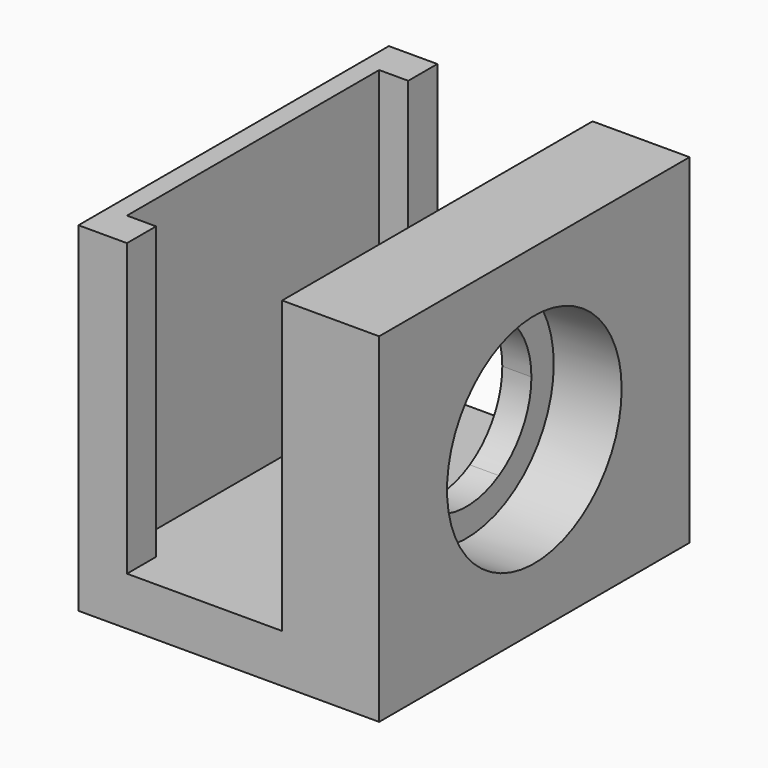
from build123d import *

# Parameters (mm, degrees)
F1_DEPTH = 20
F2_R     = 11.25
F3_DEPTH = 7
F4_R     = 6.75
F5_DEPTH = 5
F6_W     = 3
F6_H     = 32.5
F7_DEPTH = 30
F8_R     = 6.75
F9_DEPTH = 25


with BuildPart() as f1:
    # F0 (on Front) → F1 (new body, symmetric)
    with BuildSketch(Plane.XZ):
        Polygon((-25, 35), (-30, 35), (-30, 0), (1, 0), (1, 35), (-9, 35), (-9, 5), (-25, 5), align=None)
    extrude(amount=F1_DEPTH, both=True)

    # F2 (on face) → F3 (cut)
    with BuildSketch(Plane.YZ.offset(1)):
        with Locations((0, 17.5)):
            Circle(F2_R)
    extrude(amount=-F3_DEPTH, mode=Mode.SUBTRACT)

    # F4 (on face) → F5 (cut)
    with BuildSketch(Plane.YZ.offset(-6)):
        with Locations((0, 17.5)):
            Circle(F4_R)
    extrude(amount=-F5_DEPTH, mode=Mode.SUBTRACT)

    # F6 (on face) → F7 (cut)
    with BuildSketch(Plane.XY.offset(35)):
        with Locations((-26.5, 0)):
            Rectangle(F6_W, F6_H)
    extrude(amount=-F7_DEPTH, mode=Mode.SUBTRACT)

    # F8 (on face) → F9 (cut)
    with BuildSketch(Plane(origin=(-9, 0, 0), x_dir=(0, -1, 0), z_dir=(-1, 0, 0))):
        Polygon((4.1857894516, 24.75), (-4.1857894516, 24.75), (-8.3715789032, 17.5), (-4.1857894516, 10.25), (4.1857894516, 10.25), (8.3715789032, 17.5), align=None)
        with Locations((0, 17.5)):
            Circle(F8_R, mode=Mode.SUBTRACT)
        with Locations((0, 17.5)):
            Circle(F8_R)
        with BuildLine():
            ThreePointArc((4.1857894516, 24.75), (0, 25.8715789032), (-4.1857894516, 24.75))
            Line((-4.1857894516, 24.75), (4.1857894516, 24.75))
        make_face()
        with BuildLine():
            Line((-8.3715789032, 17.5), (-4.1857894516, 24.75))
            ThreePointArc((-4.1857894516, 24.75), (-7.25, 21.6857894516), (-8.3715789032, 17.5))
        make_face()
        with BuildLine():
            ThreePointArc((8.3715789032, 17.5), (7.25, 21.6857894516), (4.1857894516, 24.75))
            Line((4.1857894516, 24.75), (8.3715789032, 17.5))
        make_face()
        with BuildLine():
            Line((-4.1857894516, 10.25), (-8.3715789032, 17.5))
            ThreePointArc((-8.3715789032, 17.5), (-7.25, 13.3142105484), (-4.1857894516, 10.25))
        make_face()
        with BuildLine():
            ThreePointArc((4.1857894516, 10.25), (7.25, 13.3142105484), (8.3715789032, 17.5))
            Line((8.3715789032, 17.5), (4.1857894516, 10.25))
        make_face()
        with BuildLine():
            Line((4.1857894516, 10.25), (-4.1857894516, 10.25))
            ThreePointArc((-4.1857894516, 10.25), (0, 9.1284210968), (4.1857894516, 10.25))
        make_face()
    extrude(amount=-F9_DEPTH, mode=Mode.SUBTRACT)


solid = f1.part
